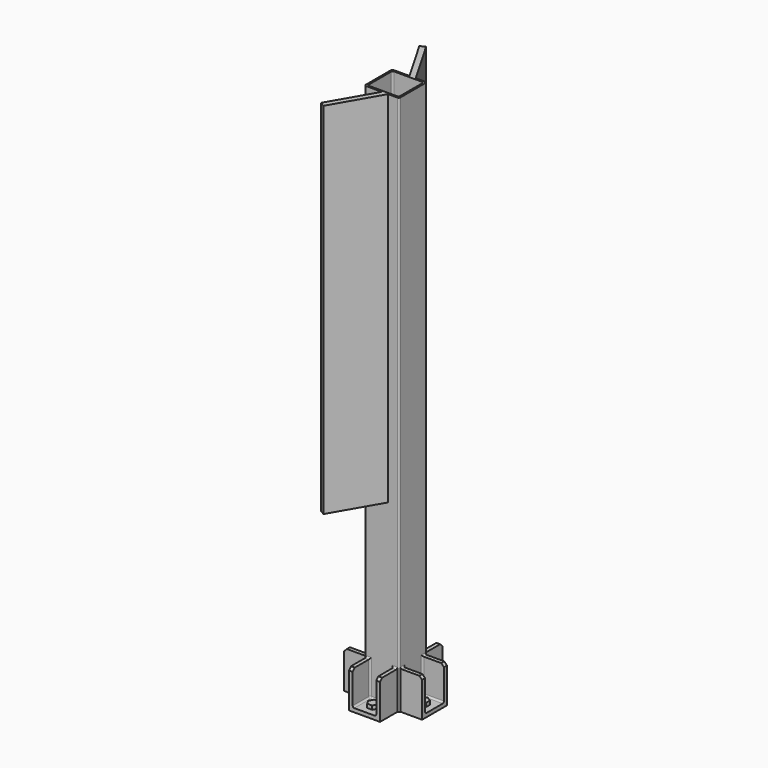
from build123d import *

# Parameters (mm, degrees)
F1_DEPTH      = 5000
F0_W          = 218
F0_H          = 200
F0_W_2        = 200
F0_H_2        = 218
F2_DEPTH      = 35
F0_W_3        = 35
F0_H_3        = 35
F3_DEPTH      = 350
F4_DEPTH      = 70
F5_SIZE       = 25
F6_T1_DEPTH   = 300
F6_T3_DEPTH   = 315
F6_T5_DEPTH   = 185
F6_T7_DEPTH   = 188
F6_T9_DEPTH   = 185
F6_T11_DEPTH  = 188
F6_T13_DEPTH  = 185
F6_T15_DEPTH  = 35
F6_T17_DEPTH  = 35
F6_T19_DEPTH  = 35
F6_T21_DEPTH  = 35
F6_S25_W      = 15.3
F6_S25_H      = 15.3
F6_T26_DEPTH  = 15.3
F6_S31_W      = 15.3
F6_S31_H      = 15.3
F6_T32_DEPTH  = 15.3
F6_S37_W      = 15.3
F6_S37_H      = 15.3
F6_T38_DEPTH  = 15.3
F6_S43_W      = 15.3
F6_S43_H      = 15.3
F6_T44_DEPTH  = 15.3
F6_S49_W      = 15.3
F6_S49_H      = 15.3
F6_T50_DEPTH  = 15.3
F6_S55_W      = 15.3
F6_S55_H      = 15.3
F6_T56_DEPTH  = 15.3
F6_T62_DEPTH  = 237.5
F6_T67_DEPTH  = 237.5
F6_T73_DEPTH  = 72.5
F6_T77_DEPTH  = 337.5
F6_T84_DEPTH  = 337.5
F6_T88_DEPTH  = 72.5
F6_T95_DEPTH  = 337.5
F6_T99_DEPTH  = 72.5
F6_T106_DEPTH = 72.5
F6_T110_DEPTH = 337.5
F6_T117_DEPTH = 337.5
F6_T121_DEPTH = 72.5
F6_T128_DEPTH = 352.5
F6_T132_DEPTH = 72.5
F6_T139_DEPTH = 72.5
F6_T143_DEPTH = 337.5
F6_T150_DEPTH = 72.5
F6_T154_DEPTH = 352.5
F7_W          = 100
F7_H          = 250
F7_W_2        = 88
F8_DEPTH      = 100
F10_DEPTH     = 288
F12_DEPTH     = 2723
F14_DEPTH     = 3323


# Not quite as in the source:
# - a fillet or chamfer that OpenCascade refuses, or shapes differently, is made with other operations: its cross-section is extruded or revolved along the edge and cut away or added


with BuildPart() as f1:
    # F0 (on Top) → F1 (new body)
    with BuildSketch(Plane.XY):
        with BuildLine():
            Line((109, -160), (144, -160))
            ThreePointArc((144, -160), (155.313708499, -155.313708499), (160, -144))
            Line((160, -144), (160, -109))
            Line((160, -109), (160, 109))
            Line((160, 109), (160, 144))
            ThreePointArc((160, 144), (155.313708499, 155.313708499), (144, 160))
            Line((144, 160), (109, 160))
            Line((109, 160), (-109, 160))
            Line((-109, 160), (-144, 160))
            ThreePointArc((-144, 160), (-155.313708499, 155.313708499), (-160, 144))
            Line((-160, 144), (-160, 109))
            Line((-160, 109), (-160, -109))
            Line((-160, -109), (-160, -144))
            ThreePointArc((-160, -144), (-155.313708499, -155.313708499), (-144, -160))
            Line((-144, -160), (-109, -160))
            Line((-109, -160), (109, -160))
        make_face()
        with BuildLine():
            Line((-128, 144), (128, 144))
            ThreePointArc((128, 144), (139.313708499, 139.313708499), (144, 128))
            Line((144, 128), (144, -128))
            ThreePointArc((144, -128), (139.313708499, -139.313708499), (128, -144))
            Line((128, -144), (-128, -144))
            ThreePointArc((-128, -144), (-139.313708499, -139.313708499), (-144, -128))
            Line((-144, -128), (-144, 128))
            ThreePointArc((-144, 128), (-139.313708499, 139.313708499), (-128, 144))
        make_face(mode=Mode.SUBTRACT)
    extrude(amount=F1_DEPTH)

    # F0 (on Top) → F2 (join)
    with BuildSketch(Plane.XY):
        with Locations((0, 260)):
            Rectangle(F0_W, F0_H)
        Polygon((23.2698549147, 299.8979596669), (46.1875740881, 259.7966943349), (22.9177191733, 219.898734668), (-23.2698549147, 220.1020403331), (-46.1875740881, 260.2033056651), (-22.9177191733, 300.101265332), align=None, mode=Mode.SUBTRACT)
        with Locations((260, 0)):
            Rectangle(F0_W_2, F0_H_2)
        Polygon((260.2033056651, 46.1875740881), (300.101265332, 22.9177191733), (299.8979596669, -23.2698549147), (259.7966943349, -46.1875740881), (219.898734668, -22.9177191733), (220.1020403331, 23.2698549147), align=None, mode=Mode.SUBTRACT)
        with Locations((0, -260)):
            Rectangle(F0_W, F0_H)
        Polygon((46.1875740881, -260.2033056651), (22.9177191733, -300.101265332), (-23.2698549147, -299.8979596669), (-46.1875740881, -259.7966943349), (-22.9177191733, -219.898734668), (23.2698549147, -220.1020403331), align=None, mode=Mode.SUBTRACT)
        with Locations((-260, 0)):
            Rectangle(F0_W_2, F0_H_2)
        Polygon((-260.2033056651, -46.1875740881), (-300.101265332, -22.9177191733), (-299.8979596669, 23.2698549147), (-259.7966943349, 46.1875740881), (-219.898734668, 22.9177191733), (-220.1020403331, -23.2698549147), align=None, mode=Mode.SUBTRACT)
    extrude(amount=F2_DEPTH)

    # F0 (on Top) → F3 (join)
    with BuildSketch(Plane.XY):
        with Locations((-126.5, 260)):
            Rectangle(F0_W_3, F0_H)
        with Locations((126.5, 260)):
            Rectangle(F0_W_3, F0_H)
        with Locations((260, 126.5)):
            Rectangle(F0_W_2, F0_H_3)
        with Locations((260, -126.5)):
            Rectangle(F0_W_2, F0_H_3)
        with Locations((126.5, -260)):
            Rectangle(F0_W_3, F0_H)
        with Locations((-260, -126.5)):
            Rectangle(F0_W_2, F0_H_3)
        with Locations((-260, 126.5)):
            Rectangle(F0_W_2, F0_H_3)
        with Locations((-126.5, -260)):
            Rectangle(F0_W_3, F0_H)
    extrude(amount=F3_DEPTH)

    # F0 (on Top) → F4 (join, through all)
    with BuildSketch(Plane.XY):
        Polygon((-299.8979596669, 23.2698549147), (-300.101265332, -22.9177191733), (-260.2033056651, -46.1875740881), (-220.1020403331, -23.2698549147), (-219.898734668, 22.9177191733), (-259.7966943349, 46.1875740881), align=None)
        Polygon((-23.2698549147, -299.8979596669), (22.9177191733, -300.101265332), (46.1875740881, -260.2033056651), (23.2698549147, -220.1020403331), (-22.9177191733, -219.898734668), (-46.1875740881, -259.7966943349), align=None)
        Polygon((299.8979596669, -23.2698549147), (300.101265332, 22.9177191733), (260.2033056651, 46.1875740881), (220.1020403331, 23.2698549147), (219.898734668, -22.9177191733), (259.7966943349, -46.1875740881), align=None)
        Polygon((22.9177191733, 219.898734668), (46.1875740881, 259.7966943349), (23.2698549147, 299.8979596669), (-22.9177191733, 300.101265332), (-46.1875740881, 260.2033056651), (-23.2698549147, 220.1020403331), align=None)
    extrude(amount=F4_DEPTH)

    # F5
    f5_edges = [f1.edges().sort_by_distance(p)[0] for p in [
        (126.5, -360, 350),
        (-126.5, -360, 350),
        (-360, 126.5, 350),
        (-360, -126.5, 350),
        (126.5, 360, 350),
        (-126.5, 360, 350),
        (360, -126.5, 350),
        (360, 126.5, 350),
    ]]
    chamfer(f5_edges, length=F5_SIZE)

    # F6: fillet of radius 15 on 27 edges, made by hand

    # F6_s2 → F6_t1 (join)
    with BuildSketch(Plane.XY.offset(50)):
        with BuildLine():
            ThreePointArc((160, -94), (164.3933982822, -104.6066017178), (175, -109))
            Line((175, -109), (160, -109))
            Line((160, -109), (160, -94))
        make_face()
        with BuildLine():
            ThreePointArc((-94, 160), (-104.6066017178, 164.3933982822), (-109, 175))
            Line((-109, 175), (-109, 160))
            Line((-109, 160), (-94, 160))
        make_face()
        with BuildLine():
            ThreePointArc((160, 94), (164.3933982822, 104.6066017178), (175, 109))
            Line((175, 109), (160, 109))
            Line((160, 109), (160, 94))
        make_face()
        with BuildLine():
            ThreePointArc((-109, -175), (-104.6066017178, -164.3933982822), (-94, -160))
            Line((-94, -160), (-109, -160))
            Line((-109, -160), (-109, -175))
        make_face()
        with BuildLine():
            ThreePointArc((94, -160), (104.6066017178, -164.3933982822), (109, -175))
            Line((109, -175), (109, -160))
            Line((109, -160), (94, -160))
        make_face()
        with BuildLine():
            ThreePointArc((94, 160), (104.6066017178, 164.3933982822), (109, 175))
            Line((109, 175), (109, 160))
            Line((109, 160), (94, 160))
        make_face()
    extrude(amount=F6_T1_DEPTH)

    # F6_s4 → F6_t3 (join)
    with BuildSketch(Plane.XY.offset(35)):
        with BuildLine():
            ThreePointArc((-160, -94), (-164.3933982822, -104.6066017178), (-175, -109))
            Line((-175, -109), (-160, -109))
            Line((-160, -109), (-160, -94))
        make_face()
        with BuildLine():
            ThreePointArc((-160, 94), (-164.3933982822, 104.6066017178), (-175, 109))
            Line((-175, 109), (-160, 109))
            Line((-160, 109), (-160, 94))
        make_face()
    extrude(amount=F6_T3_DEPTH)

    # F6_s6 → F6_t5 (join)
    with BuildSketch(Plane.XZ.offset(-360)):
        with BuildLine():
            ThreePointArc((-94, 35), (-104.6066017178, 39.3933982822), (-109, 50))
            Line((-109, 50), (-109, 35))
            Line((-109, 35), (-94, 35))
        make_face()
        with BuildLine():
            ThreePointArc((109, 50), (104.6066017178, 39.3933982822), (94, 35))
            Line((94, 35), (109, 35))
            Line((109, 35), (109, 50))
        make_face()
    extrude(amount=F6_T5_DEPTH)

    # F6_s8 → F6_t7 (join)
    with BuildSketch(Plane.YZ.offset(-94)):
        with BuildLine():
            ThreePointArc((160, 50), (164.3933982822, 39.3933982822), (175, 35))
            Line((175, 35), (160, 35))
            Line((160, 35), (160, 50))
        make_face()
        with BuildLine():
            ThreePointArc((-160, 50), (-164.3933982822, 39.3933982822), (-175, 35))
            Line((-175, 35), (-160, 35))
            Line((-160, 35), (-160, 50))
        make_face()
    extrude(amount=F6_T7_DEPTH)

    # F6_s10 → F6_t9 (join)
    with BuildSketch(Plane.YZ.offset(175)):
        with BuildLine():
            ThreePointArc((94, 35), (104.6066017178, 39.3933982822), (109, 50))
            Line((109, 50), (109, 35))
            Line((109, 35), (94, 35))
        make_face()
        with BuildLine():
            ThreePointArc((-109, 50), (-104.6066017178, 39.3933982822), (-94, 35))
            Line((-94, 35), (-109, 35))
            Line((-109, 35), (-109, 50))
        make_face()
    extrude(amount=F6_T9_DEPTH)

    # F6_s12 → F6_t11 (join)
    with BuildSketch(Plane.XZ.offset(-94)):
        with BuildLine():
            ThreePointArc((160, 50), (164.3933982822, 39.3933982822), (175, 35))
            Line((175, 35), (160, 35))
            Line((160, 35), (160, 50))
        make_face()
    extrude(amount=F6_T11_DEPTH)

    # F6_s14 → F6_t13 (join)
    with BuildSketch(Plane.XZ.offset(175)):
        with BuildLine():
            ThreePointArc((94, 35), (104.6066017178, 39.3933982822), (109, 50))
            Line((109, 50), (109, 35))
            Line((109, 35), (94, 35))
        make_face()
        with BuildLine():
            ThreePointArc((-109, 50), (-104.6066017178, 39.3933982822), (-94, 35))
            Line((-94, 35), (-109, 35))
            Line((-109, 35), (-109, 50))
        make_face()
    extrude(amount=F6_T13_DEPTH)

    # F6_s16 → F6_t15 (join)
    with BuildSketch(Plane.YZ.offset(-144)):
        with BuildLine():
            ThreePointArc((-175, 350), (-164.3933982822, 354.3933982822), (-160, 365))
            Line((-160, 365), (-160, 350))
            Line((-160, 350), (-175, 350))
        make_face()
        with BuildLine():
            ThreePointArc((160, 365), (164.3933982822, 354.3933982822), (175, 350))
            Line((175, 350), (160, 350))
            Line((160, 350), (160, 365))
        make_face()
    extrude(amount=F6_T15_DEPTH)

    # F6_s18 → F6_t17 (join)
    with BuildSketch(Plane.YZ.offset(109)):
        with BuildLine():
            ThreePointArc((-160, 365), (-164.3933982822, 354.3933982822), (-175, 350))
            Line((-175, 350), (-160, 350))
            Line((-160, 350), (-160, 365))
        make_face()
        with BuildLine():
            ThreePointArc((160, 365), (164.3933982822, 354.3933982822), (175, 350))
            Line((175, 350), (160, 350))
            Line((160, 350), (160, 365))
        make_face()
    extrude(amount=F6_T17_DEPTH)

    # F6_s20 → F6_t19 (join)
    with BuildSketch(Plane.XZ.offset(109)):
        with BuildLine():
            ThreePointArc((160, 365), (164.3933982822, 354.3933982822), (175, 350))
            Line((175, 350), (160, 350))
            Line((160, 350), (160, 365))
        make_face()
        with BuildLine():
            ThreePointArc((-160, 365), (-164.3933982822, 354.3933982822), (-175, 350))
            Line((-175, 350), (-160, 350))
            Line((-160, 350), (-160, 365))
        make_face()
    extrude(amount=F6_T19_DEPTH)

    # F6_s22 → F6_t21 (join)
    with BuildSketch(Plane.XZ.offset(-144)):
        with BuildLine():
            ThreePointArc((160, 365), (164.3933982822, 354.3933982822), (175, 350))
            Line((175, 350), (160, 350))
            Line((160, 350), (160, 365))
        make_face()
        with BuildLine():
            ThreePointArc((-160, 365), (-164.3933982822, 354.3933982822), (-175, 350))
            Line((-175, 350), (-160, 350))
            Line((-160, 350), (-160, 365))
        make_face()
    extrude(amount=F6_T21_DEPTH)


with BuildPart() as f6_tool24:
    # F6_s25 → F6_t26 (new body)
    with BuildSketch(Plane.XZ.offset(94)):
        with Locations((167.35, 42.35)):
            Rectangle(F6_S25_W, F6_S25_H)
    extrude(amount=F6_T26_DEPTH)

    # F6_s27 → F6_t28 (revolve, cut)
    with BuildSketch(Plane(origin=(175, -94, 50), x_dir=(0.7071067812, 0, 0.7071067812), z_dir=(0.7071067812, 0, -0.7071067812))):
        with BuildLine():
            ThreePointArc((0, -15), (15, 0), (0, 15))
            Line((0, 15), (0, -15))
        make_face()
    revolve(axis=Axis((175, -94, 50), (0, -1, 0)), mode=Mode.SUBTRACT)


with BuildPart() as f1_1:
    add(f1.part)

    # F6_t23: union F6_tool24
    add(f6_tool24.part)


with BuildPart() as f6_tool30:
    # F6_s31 → F6_t32 (new body)
    with BuildSketch(Plane.XZ.offset(-175)):
        with Locations((-101.65, 42.35)):
            Rectangle(F6_S31_W, F6_S31_H)
    extrude(amount=F6_T32_DEPTH)

    # F6_s33 → F6_t34 (revolve, cut)
    with BuildSketch(Plane(origin=(-94, 175, 50), x_dir=(0.7071067812, 0, 0.7071067812), z_dir=(0.7071067812, 0, -0.7071067812))):
        with BuildLine():
            ThreePointArc((0, -15), (15, 0), (0, 15))
            Line((0, 15), (0, -15))
        make_face()
    revolve(axis=Axis((-94, 175, 50), (0, -1, 0)), mode=Mode.SUBTRACT)


with BuildPart() as f1_2:
    add(f1_1.part)

    # F6_t29: union F6_tool30
    add(f6_tool30.part)


with BuildPart() as f6_tool36:
    # F6_s37 → F6_t38 (new body)
    with BuildSketch(Plane.XZ.offset(-94)):
        with Locations((167.35, 42.35)):
            Rectangle(F6_S37_W, F6_S37_H)
    extrude(amount=-F6_T38_DEPTH)

    # F6_s39 → F6_t40 (revolve, cut)
    with BuildSketch(Plane(origin=(175, 94, 50), x_dir=(0.7071067812, 0, 0.7071067812), z_dir=(-0.7071067812, 0, 0.7071067812))):
        with BuildLine():
            ThreePointArc((0, -15), (15, 0), (0, 15))
            Line((0, 15), (0, -15))
        make_face()
    revolve(axis=Axis((175, 94, 50), (0, 1, 0)), mode=Mode.SUBTRACT)


with BuildPart() as f1_3:
    add(f1_2.part)

    # F6_t35: union F6_tool36
    add(f6_tool36.part)


with BuildPart() as f6_tool42:
    # F6_s43 → F6_t44 (new body)
    with BuildSketch(Plane.YZ.offset(-94)):
        with Locations((-167.35, 42.35)):
            Rectangle(F6_S43_W, F6_S43_H)
    extrude(amount=-F6_T44_DEPTH)

    # F6_s45 → F6_t46 (revolve, cut)
    with BuildSketch(Plane(origin=(-94, -175, 50), x_dir=(0, -0.7071067812, 0.7071067812), z_dir=(0, -0.7071067812, -0.7071067812))):
        with BuildLine():
            ThreePointArc((0, -15), (15, 0), (0, 15))
            Line((0, 15), (0, -15))
        make_face()
    revolve(axis=Axis((-94, -175, 50), (-1, 0, 0)), mode=Mode.SUBTRACT)


with BuildPart() as f1_4:
    add(f1_3.part)

    # F6_t41: union F6_tool42
    add(f6_tool42.part)


with BuildPart() as f6_tool48:
    # F6_s49 → F6_t50 (new body)
    with BuildSketch(Plane.YZ.offset(94)):
        with Locations((-167.35, 42.35)):
            Rectangle(F6_S49_W, F6_S49_H)
    extrude(amount=F6_T50_DEPTH)

    # F6_s51 → F6_t52 (revolve, cut)
    with BuildSketch(Plane(origin=(94, -175, 50), x_dir=(0, -0.7071067812, 0.7071067812), z_dir=(0, 0.7071067812, 0.7071067812))):
        with BuildLine():
            ThreePointArc((0, -15), (15, 0), (0, 15))
            Line((0, 15), (0, -15))
        make_face()
    revolve(axis=Axis((94, -175, 50), (1, 0, 0)), mode=Mode.SUBTRACT)


with BuildPart() as f1_5:
    add(f1_4.part)

    # F6_t47: union F6_tool48
    add(f6_tool48.part)


with BuildPart() as f6_tool54:
    # F6_s55 → F6_t56 (new body)
    with BuildSketch(Plane.XZ.offset(-175)):
        with Locations((101.65, 42.35)):
            Rectangle(F6_S55_W, F6_S55_H)
    extrude(amount=F6_T56_DEPTH)

    # F6_s57 → F6_t58 (revolve, cut)
    with BuildSketch(Plane(origin=(94, 175, 50), x_dir=(-0.7071067812, 0, 0.7071067812), z_dir=(0.7071067812, 0, 0.7071067812))):
        with BuildLine():
            ThreePointArc((0, -15), (15, 0), (0, 15))
            Line((0, 15), (0, -15))
        make_face()
    revolve(axis=Axis((94, 175, 50), (0, -1, 0)), mode=Mode.SUBTRACT)


with BuildPart() as f1_6:
    add(f1_5.part)

    # F6_t53: union F6_tool54
    add(f6_tool54.part)


with BuildPart() as f6_tool60:
    # F6_s61 → F6_t62 (new body)
    with BuildSketch(Plane.YZ.offset(-122.5)):
        with BuildLine():
            ThreePointArc((109, 50), (104.6066017178, 39.3933982822), (94, 35))
            Line((94, 35), (109, 35))
            Line((109, 35), (109, 50))
        make_face()
    extrude(amount=-F6_T62_DEPTH)

    split(bisect_by=Plane.YZ.offset(-144), keep=Keep.BOTTOM)


with BuildPart() as f1_7:
    add(f1_6.part)

    # F6_t59: union F6_tool60
    add(f6_tool60.part)


with BuildPart() as f6_tool65:
    # F6_s66 → F6_t67 (new body)
    with BuildSketch(Plane.YZ.offset(-360)):
        with BuildLine():
            ThreePointArc((-94, 35), (-104.6066017178, 39.3933982822), (-109, 50))
            Line((-109, 50), (-109, 35))
            Line((-109, 35), (-94, 35))
        make_face()
    extrude(amount=F6_T67_DEPTH)

    split(bisect_by=Plane.YZ.offset(-144), keep=Keep.BOTTOM)


with BuildPart() as f1_8:
    add(f1_7.part)

    # F6_t64: union F6_tool65
    add(f6_tool65.part)


with BuildPart() as f6_tool71:
    # F6_s72 → F6_t73 (new body)
    with BuildSketch(Plane.XZ.offset(71.5)):
        with BuildLine():
            ThreePointArc((160, 365), (164.3933982822, 354.3933982822), (175, 350))
            Line((175, 350), (160, 350))
            Line((160, 350), (160, 365))
        make_face()
    extrude(amount=F6_T73_DEPTH)

    split(bisect_by=Plane.XZ.offset(109), keep=Keep.BOTTOM)


with BuildPart() as f6_tool75:
    # F6_s76 → F6_t77 (new body)
    with BuildSketch(Plane.XY.offset(50)):
        with BuildLine():
            ThreePointArc((160, -94), (164.3933982822, -104.6066017178), (175, -109))
            Line((175, -109), (160, -109))
            Line((160, -109), (160, -94))
        make_face()
    extrude(amount=F6_T77_DEPTH)

    split(bisect_by=Plane.XY.offset(350), keep=Keep.TOP)


with BuildPart() as f6_tool71_1:
    add(f6_tool71.part)

    # F6_t79: intersect F6_tool75
    add(f6_tool75.part, mode=Mode.INTERSECT)


with BuildPart() as f1_9:
    add(f1_8.part)

    # F6_t69: union F6_tool71
    add(f6_tool71_1.part)


with BuildPart() as f6_tool82:
    # F6_s83 → F6_t84 (new body)
    with BuildSketch(Plane.XY.offset(50)):
        with BuildLine():
            ThreePointArc((-94, 160), (-104.6066017178, 164.3933982822), (-109, 175))
            Line((-109, 175), (-109, 160))
            Line((-109, 160), (-94, 160))
        make_face()
    extrude(amount=F6_T84_DEPTH)

    split(bisect_by=Plane.XY.offset(350), keep=Keep.TOP)


with BuildPart() as f6_tool86:
    # F6_s87 → F6_t88 (new body)
    with BuildSketch(Plane.YZ.offset(-144)):
        with BuildLine():
            ThreePointArc((160, 365), (164.3933982822, 354.3933982822), (175, 350))
            Line((175, 350), (160, 350))
            Line((160, 350), (160, 365))
        make_face()
    extrude(amount=F6_T88_DEPTH)

    split(bisect_by=Plane.YZ.offset(-109), keep=Keep.TOP)


with BuildPart() as f6_tool82_1:
    add(f6_tool82.part)

    # F6_t90: intersect F6_tool86
    add(f6_tool86.part, mode=Mode.INTERSECT)


with BuildPart() as f1_10:
    add(f1_9.part)

    # F6_t80: union F6_tool82
    add(f6_tool82_1.part)


with BuildPart() as f6_tool93:
    # F6_s94 → F6_t95 (new body)
    with BuildSketch(Plane.XY.offset(50)):
        with BuildLine():
            ThreePointArc((160, 94), (164.3933982822, 104.6066017178), (175, 109))
            Line((175, 109), (160, 109))
            Line((160, 109), (160, 94))
        make_face()
    extrude(amount=F6_T95_DEPTH)

    split(bisect_by=Plane.XY.offset(350), keep=Keep.TOP)


with BuildPart() as f6_tool97:
    # F6_s98 → F6_t99 (new body)
    with BuildSketch(Plane.XZ.offset(-144)):
        with BuildLine():
            ThreePointArc((160, 365), (164.3933982822, 354.3933982822), (175, 350))
            Line((175, 350), (160, 350))
            Line((160, 350), (160, 365))
        make_face()
    extrude(amount=F6_T99_DEPTH)

    split(bisect_by=Plane.XZ.offset(-109), keep=Keep.TOP)


with BuildPart() as f6_tool93_1:
    add(f6_tool93.part)

    # F6_t101: intersect F6_tool97
    add(f6_tool97.part, mode=Mode.INTERSECT)


with BuildPart() as f1_11:
    add(f1_10.part)

    # F6_t91: union F6_tool93
    add(f6_tool93_1.part)


with BuildPart() as f6_tool104:
    # F6_s105 → F6_t106 (new body)
    with BuildSketch(Plane.YZ.offset(-71.5)):
        with BuildLine():
            ThreePointArc((-175, 350), (-164.3933982822, 354.3933982822), (-160, 365))
            Line((-160, 365), (-160, 350))
            Line((-160, 350), (-175, 350))
        make_face()
    extrude(amount=-F6_T106_DEPTH)

    split(bisect_by=Plane.YZ.offset(-109), keep=Keep.TOP)


with BuildPart() as f6_tool108:
    # F6_s109 → F6_t110 (new body)
    with BuildSketch(Plane.XY.offset(50)):
        with BuildLine():
            ThreePointArc((-109, -175), (-104.6066017178, -164.3933982822), (-94, -160))
            Line((-94, -160), (-109, -160))
            Line((-109, -160), (-109, -175))
        make_face()
    extrude(amount=F6_T110_DEPTH)

    split(bisect_by=Plane.XY.offset(350), keep=Keep.TOP)


with BuildPart() as f6_tool104_1:
    add(f6_tool104.part)

    # F6_t112: intersect F6_tool108
    add(f6_tool108.part, mode=Mode.INTERSECT)


with BuildPart() as f1_12:
    add(f1_11.part)

    # F6_t102: union F6_tool104
    add(f6_tool104_1.part)


with BuildPart() as f6_tool115:
    # F6_s116 → F6_t117 (new body)
    with BuildSketch(Plane.XY.offset(50)):
        with BuildLine():
            ThreePointArc((94, -160), (104.6066017178, -164.3933982822), (109, -175))
            Line((109, -175), (109, -160))
            Line((109, -160), (94, -160))
        make_face()
    extrude(amount=F6_T117_DEPTH)

    split(bisect_by=Plane.XY.offset(350), keep=Keep.TOP)


with BuildPart() as f6_tool119:
    # F6_s120 → F6_t121 (new body)
    with BuildSketch(Plane.YZ.offset(144)):
        with BuildLine():
            ThreePointArc((-160, 365), (-164.3933982822, 354.3933982822), (-175, 350))
            Line((-175, 350), (-160, 350))
            Line((-160, 350), (-160, 365))
        make_face()
    extrude(amount=-F6_T121_DEPTH)

    split(bisect_by=Plane.YZ.offset(109), keep=Keep.BOTTOM)


with BuildPart() as f6_tool115_1:
    add(f6_tool115.part)

    # F6_t123: intersect F6_tool119
    add(f6_tool119.part, mode=Mode.INTERSECT)


with BuildPart() as f1_13:
    add(f1_12.part)

    # F6_t113: union F6_tool115
    add(f6_tool115_1.part)


with BuildPart() as f6_tool126:
    # F6_s127 → F6_t128 (new body)
    with BuildSketch(Plane.XY.offset(35)):
        with BuildLine():
            ThreePointArc((-160, -94), (-164.3933982822, -104.6066017178), (-175, -109))
            Line((-175, -109), (-160, -109))
            Line((-160, -109), (-160, -94))
        make_face()
    extrude(amount=F6_T128_DEPTH)

    split(bisect_by=Plane.XY.offset(350), keep=Keep.TOP)


with BuildPart() as f6_tool130:
    # F6_s131 → F6_t132 (new body)
    with BuildSketch(Plane.XZ.offset(144)):
        with BuildLine():
            ThreePointArc((-160, 365), (-164.3933982822, 354.3933982822), (-175, 350))
            Line((-175, 350), (-160, 350))
            Line((-160, 350), (-160, 365))
        make_face()
    extrude(amount=-F6_T132_DEPTH)

    split(bisect_by=Plane.XZ.offset(109), keep=Keep.BOTTOM)


with BuildPart() as f6_tool126_1:
    add(f6_tool126.part)

    # F6_t134: intersect F6_tool130
    add(f6_tool130.part, mode=Mode.INTERSECT)


with BuildPart() as f1_14:
    add(f1_13.part)

    # F6_t124: union F6_tool126
    add(f6_tool126_1.part)


with BuildPart() as f6_tool137:
    # F6_s138 → F6_t139 (new body)
    with BuildSketch(Plane.YZ.offset(71.5)):
        with BuildLine():
            ThreePointArc((160, 365), (164.3933982822, 354.3933982822), (175, 350))
            Line((175, 350), (160, 350))
            Line((160, 350), (160, 365))
        make_face()
    extrude(amount=F6_T139_DEPTH)

    split(bisect_by=Plane.YZ.offset(109), keep=Keep.BOTTOM)


with BuildPart() as f6_tool141:
    # F6_s142 → F6_t143 (new body)
    with BuildSketch(Plane.XY.offset(50)):
        with BuildLine():
            ThreePointArc((94, 160), (104.6066017178, 164.3933982822), (109, 175))
            Line((109, 175), (109, 160))
            Line((109, 160), (94, 160))
        make_face()
    extrude(amount=F6_T143_DEPTH)

    split(bisect_by=Plane.XY.offset(350), keep=Keep.TOP)


with BuildPart() as f6_tool137_1:
    add(f6_tool137.part)

    # F6_t145: intersect F6_tool141
    add(f6_tool141.part, mode=Mode.INTERSECT)


with BuildPart() as f1_15:
    add(f1_14.part)

    # F6_t135: union F6_tool137
    add(f6_tool137_1.part)


with BuildPart() as f6_tool148:
    # F6_s149 → F6_t150 (new body)
    with BuildSketch(Plane.XZ.offset(-71.5)):
        with BuildLine():
            ThreePointArc((-160, 365), (-164.3933982822, 354.3933982822), (-175, 350))
            Line((-175, 350), (-160, 350))
            Line((-160, 350), (-160, 365))
        make_face()
    extrude(amount=-F6_T150_DEPTH)

    split(bisect_by=Plane.XZ.offset(-109), keep=Keep.TOP)


with BuildPart() as f6_tool152:
    # F6_s153 → F6_t154 (new body)
    with BuildSketch(Plane.XY.offset(35)):
        with BuildLine():
            ThreePointArc((-160, 94), (-164.3933982822, 104.6066017178), (-175, 109))
            Line((-175, 109), (-160, 109))
            Line((-160, 109), (-160, 94))
        make_face()
    extrude(amount=F6_T154_DEPTH)

    split(bisect_by=Plane.XY.offset(350), keep=Keep.TOP)


with BuildPart() as f6_tool148_1:
    add(f6_tool148.part)

    # F6_t156: intersect F6_tool152
    add(f6_tool152.part, mode=Mode.INTERSECT)


with BuildPart() as f1_16:
    add(f1_15.part)

    # F6_t146: union F6_tool148
    add(f6_tool148_1.part)

    # F7 (on face) → F8 (join)
    with BuildSketch(Plane(origin=(-160, 0, 0), x_dir=(0, -1, 0), z_dir=(-1, 0, 0))):
        with Locations((-94, 4275)):
            Rectangle(F7_W, F7_H)
        with Locations((-94, 4025)):
            Rectangle(F7_W, F7_H)
        with Locations((94, 4275)):
            Rectangle(F7_W, F7_H)
        with Locations((94, 4025)):
            Rectangle(F7_W, F7_H)
        with Locations((-94, 2052)):
            Rectangle(F7_W, F7_H)
        with Locations((-94, 1802)):
            Rectangle(F7_W, F7_H)
        with Locations((94, 2052)):
            Rectangle(F7_W, F7_H)
        with Locations((94, 1802)):
            Rectangle(F7_W, F7_H)
        with Locations((0, 4275)):
            Rectangle(F7_W_2, F7_H)
        with Locations((0, 4025)):
            Rectangle(F7_W_2, F7_H)
        with Locations((0, 2052)):
            Rectangle(F7_W_2, F7_H)
        with Locations((0, 1802)):
            Rectangle(F7_W_2, F7_H)
    extrude(amount=F8_DEPTH)

    # F9 (on face) → F10 (join, through all)
    with BuildSketch(Plane.XZ.offset(144)):
        with BuildLine():
            Line((-270.811035037, 4150), (-260, 4150))
            Line((-260, 4150), (-260, 4353.9996147156))
            ThreePointArc((-260, 4353.9996147156), (-294.1870067447, 4279.8901495486), (-370.1304380318, 4249.9976839118))
            ThreePointArc((-370.1304380318, 4249.9976839118), (-299.8601375779, 4220.4696399149), (-270.811035037, 4150))
        make_face()
        with BuildLine():
            Line((-320.811035037, 4150), (-270.811035037, 4150))
            ThreePointArc((-270.811035037, 4150), (-299.8601375779, 4220.4696399149), (-370.1304380318, 4249.9976839118))
            ThreePointArc((-370.1304380318, 4249.9976839118), (-441.2806749519, 4220.9508974592), (-470.811035037, 4150))
            Line((-470.811035037, 4150), (-420.811035037, 4150))
            ThreePointArc((-420.811035037, 4150), (-370.811035037, 4200), (-320.811035037, 4150))
        make_face()
        with BuildLine():
            ThreePointArc((-365.8744445903, 4050.1219239534), (-298.3760329846, 4081.0567590139), (-270.811035037, 4150))
            Line((-270.811035037, 4150), (-320.811035037, 4150))
            ThreePointArc((-320.811035037, 4150), (-370.811035037, 4100), (-420.811035037, 4150))
            Line((-420.811035037, 4150), (-470.811035037, 4150))
            ThreePointArc((-470.811035037, 4150), (-439.7542760231, 4077.5649979475), (-365.8744445903, 4050.1219239534))
        make_face()
        with BuildLine():
            Line((-260, 3959.3045621135), (-260, 4150))
            Line((-260, 4150), (-270.811035037, 4150))
            ThreePointArc((-270.811035037, 4150), (-298.3760329846, 4081.0567590139), (-365.8744445903, 4050.1219239534))
            ThreePointArc((-365.8744445903, 4050.1219239534), (-294.8430129594, 4025.807385441), (-260, 3959.3045621135))
        make_face()
        with BuildLine():
            Line((-320.3974096751, 1913.7505576502), (-270.3974096751, 1913.7505576502))
            ThreePointArc((-270.3974096751, 1913.7505576502), (-299.5256261389, 1984.2997624537), (-369.9412156431, 2013.7495170798))
            ThreePointArc((-369.9412156431, 2013.7495170798), (-440.9466144785, 1984.6223411864), (-470.3974096751, 1913.7505576502))
            Line((-470.3974096751, 1913.7505576502), (-420.3974096751, 1913.7505576502))
            ThreePointArc((-420.3974096751, 1913.7505576502), (-370.3974096751, 1963.7505576502), (-320.3974096751, 1913.7505576502))
        make_face()
        with BuildLine():
            ThreePointArc((-365.4608192283, 1813.8724816036), (-297.9624076226, 1844.8073166641), (-270.3974096751, 1913.7505576502))
            Line((-270.3974096751, 1913.7505576502), (-320.3974096751, 1913.7505576502))
            ThreePointArc((-320.3974096751, 1913.7505576502), (-370.3974096751, 1863.7505576502), (-420.3974096751, 1913.7505576502))
            Line((-420.3974096751, 1913.7505576502), (-470.3974096751, 1913.7505576502))
            ThreePointArc((-470.3974096751, 1913.7505576502), (-439.3406506611, 1841.3155555977), (-365.4608192283, 1813.8724816036))
        make_face()
        with BuildLine():
            Line((-260, 1726.4739451434), (-260, 1913.7505576502))
            Line((-260, 1913.7505576502), (-270.3974096751, 1913.7505576502))
            ThreePointArc((-270.3974096751, 1913.7505576502), (-297.9624076226, 1844.8073166641), (-365.4608192283, 1813.8724816036))
            ThreePointArc((-365.4608192283, 1813.8724816036), (-295.7458390107, 1790.6679127429), (-260, 1726.4739451434))
        make_face()
        with BuildLine():
            Line((-270.3974096751, 1913.7505576502), (-260, 1913.7505576502))
            Line((-260, 1913.7505576502), (-260, 2119.0190959001))
            ThreePointArc((-260, 2119.0190959001), (-293.6952390113, 2044.1647827067), (-369.9412156431, 2013.7495170798))
            ThreePointArc((-369.9412156431, 2013.7495170798), (-299.5256261389, 1984.2997624537), (-270.3974096751, 1913.7505576502))
        make_face()
    extrude(amount=-F10_DEPTH)

    # F11 (on face) → F12 (cut, through all)
    with BuildSketch(Plane.XY.offset(4400)):
        Polygon((-470.811035037, 75), (-470.811035037, 0), (-470.811035037, -75), (-260, -75), (-260, 75), align=None)
    extrude(amount=-F12_DEPTH, mode=Mode.SUBTRACT)

    # F13 (on face) → F14 (join, through all)
    with BuildSketch(Plane.XY.offset(5000)):
        Polygon((0, 160), (57.735026919, 160), (-192.264973081, 593.0127018922), (-235.5662432703, 568.0127018922), align=None)
        Polygon((-192.264973081, -593.0127018922), (57.735026919, -160), (0, -160), (-235.5662432703, -568.0127018922), align=None)
    extrude(amount=-F14_DEPTH)


solid = f1_16.part
